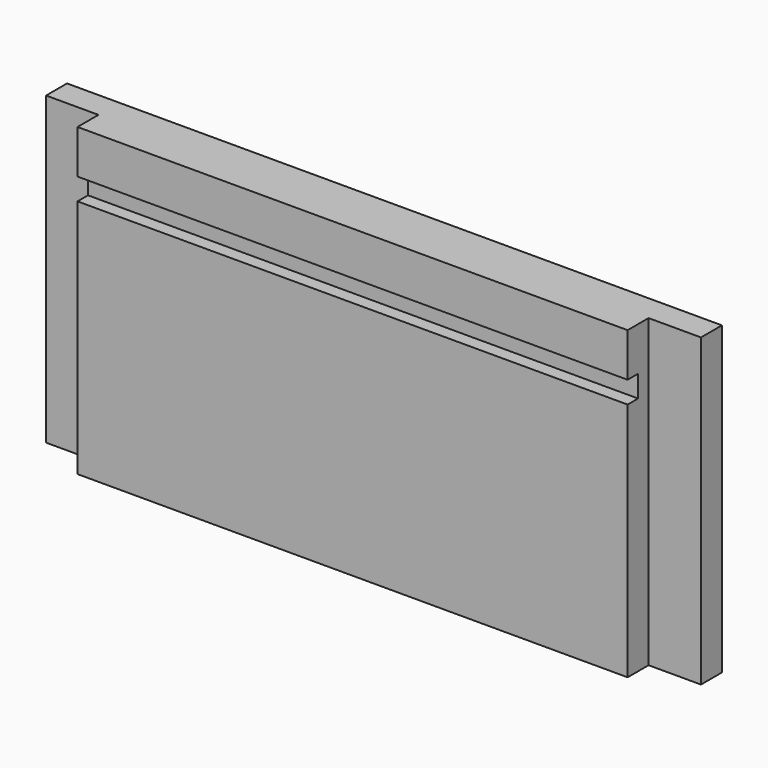
from build123d import *

# Parameters (mm, degrees)
F1_DEPTH = 150
F2_W     = 12
F2_H     = 70
F3_DEPTH = 6


# Not quite as in the source:
# - a feature names something its author has since deleted; it is built from what else it names


with BuildPart() as f1:
    # F0 (on Right) → F1 (new body)
    with BuildSketch(Plane.YZ):
        Polygon((-12, 0), (0, 0), (0, 70), (-12, 70), (-12, 60), (-9, 60), (-9, 55), (-12, 55), align=None)
    extrude(amount=F1_DEPTH)

    # F2 (on face) → F3 (cut)
    with BuildSketch(Plane.XZ.offset(12)):
        with Locations((144, 35)):
            Rectangle(F2_W, F2_H)
        with Locations((6, 35)):
            Rectangle(F2_W, F2_H)
    extrude(amount=-F3_DEPTH, mode=Mode.SUBTRACT)


solid = f1.part
